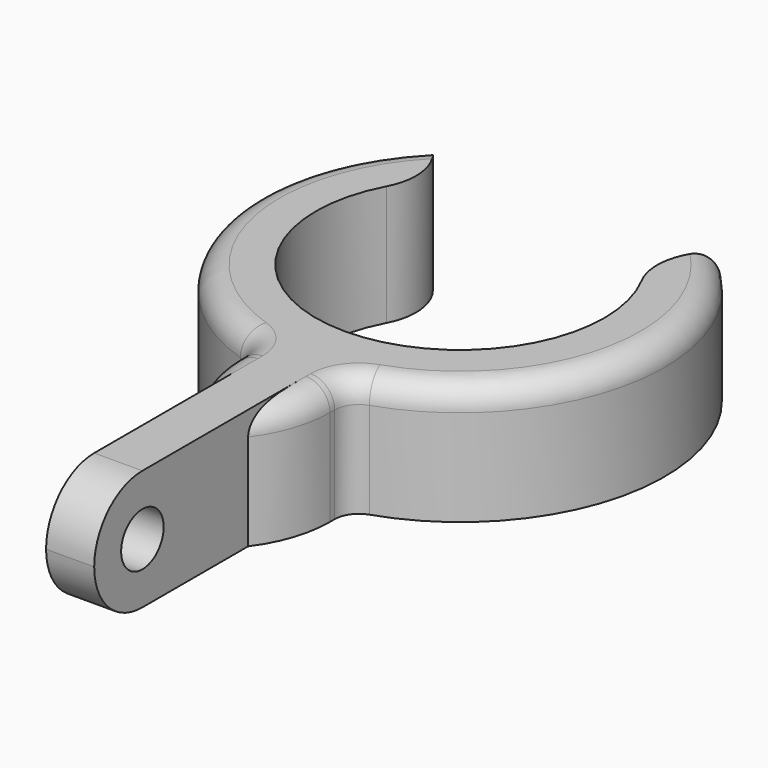
from build123d import *

# Parameters (mm, degrees)
F1_DEPTH    = 5
F2_R        = 1.1043953889
F3_DEPTH    = 5
F4_R        = 2.5
F5_T1_DEPTH = 20
F6_F1_R     = 1
F6_F2_R     = 1
F6_F3_R     = 0.9999
F6_F4_R     = 0.9996
F7_R        = 2.49999


# Not quite as in the source:
# - a fillet or chamfer that OpenCascade refuses, or shapes differently, is made with other operations: its cross-section is extruded or revolved along the edge and cut away or added
# - a fillet or chamfer is up to 0.001 mm smaller than in the source, because OpenCascade refuses the exact size


with BuildPart() as f1:
    # F0 (on Top) → F1 (new body)
    with BuildSketch(Plane.XY):
        with BuildLine():
            ThreePointArc((4.2426406871, 4.2426406871), (0, -6), (-4.2426406871, 4.2426406871))
            Line((-4.2426406871, 4.2426406871), (-6.0104076401, 6.0104076401))
            ThreePointArc((-6.0104076401, 6.0104076401), (-8.1830596791, -2.2994639132), (-2, -8.2613558209))
            Line((-2, -8.2613558209), (-2, -12.2613558209))
            Line((-2, -12.2613558209), (-1, -12.2613558209))
            Line((-1, -12.2613558209), (-1, -20.2613558209))
            Line((-1, -20.2613558209), (0, -20.2613558209))
            Line((0, -20.2613558209), (1, -20.2613558209))
            Line((1, -20.2613558209), (1, -12.2613558209))
            Line((1, -12.2613558209), (2, -12.2613558209))
            Line((2, -12.2613558209), (2, -8.2613558209))
            ThreePointArc((2, -8.2613558209), (8.1830596791, -2.2994639132), (6.0104076401, 6.0104076401))
            Line((6.0104076401, 6.0104076401), (4.2426406871, 4.2426406871))
        make_face()
    extrude(amount=F1_DEPTH)

    # F2 (on face) → F3 (cut)
    with BuildSketch(Plane(origin=(-1, 0, 0), x_dir=(0, -1, 0), z_dir=(-1, 0, 0))):
        with Locations((17.756960432, 2.4956046111)):
            Circle(F2_R)
    extrude(amount=-F3_DEPTH, mode=Mode.SUBTRACT)

    # F4
    f4_edges = [f1.edges().sort_by_distance(p)[0] for p in [
        (4.242641, 4.242641, 2.5),
        (-4.242641, 4.242641, 2.5),
    ]]
    fillet(f4_edges, radius=F4_R)

    # F5: fillet of radius 5 on 2 edges, made by hand

    # F5_s2 → F5_t1 (cut)
    with BuildSketch(Plane.XY.offset(-7.5)):
        with BuildLine():
            ThreePointArc((2, -9.2613558209), (1.7434164903, -10.842494651), (1, -12.2613558209))
            Line((1, -12.2613558209), (2, -12.2613558209))
            Line((2, -12.2613558209), (2, -9.2613558209))
        make_face()
        with BuildLine():
            ThreePointArc((-2, -9.2613558209), (-1.7434164903, -10.842494651), (-1, -12.2613558209))
            Line((-1, -12.2613558209), (-2, -12.2613558209))
            Line((-2, -12.2613558209), (-2, -9.2613558209))
        make_face()
    extrude(amount=F5_T1_DEPTH, mode=Mode.SUBTRACT)

    # F6: fillet of radius 1 on 6 edges, made by hand

    # F6_f1
    f6_f1_edges = [f1.edges().sort_by_distance(p)[0] for p in [
        (-2, -8.2613558209, 2.5),
    ]]
    fillet(f6_f1_edges, radius=F6_F1_R)

    # F6_f2
    f6_f2_edges = [f1.edges().sort_by_distance(p)[0] for p in [
        (2, -8.2613558209, 2.5),
    ]]
    fillet(f6_f2_edges, radius=F6_F2_R)

    # F6_f3 (radius 1 in the source; OpenCascade refuses exactly that, so slightly less here)
    f6_f3_edges = [f1.edges().sort_by_distance(p)[0] for p in [
        (2, -9.1376170048, 5),
        (1.7434164903, -10.842494651, 5),
    ]]
    fillet(f6_f3_edges, radius=F6_F3_R)

    # F6_f4 (radius 1 in the source; OpenCascade refuses exactly that, so slightly less here)
    f6_f4_edges = [f1.edges().sort_by_distance(p)[0] for p in [
        (-1.7434164903, -10.842494651, 5),
        (-2, -9.1376170048, 5),
    ]]
    fillet(f6_f4_edges, radius=F6_F4_R)

    # F7 (radius 2.5 in the source; OpenCascade refuses exactly that, so slightly less here)
    f7_edges = [f1.edges().sort_by_distance(p)[0] for p in [
        (0, -20.261356, 5),
        (0, -20.261356, 0),
    ]]
    fillet(f7_edges, radius=F7_R)


solid = f1.part
